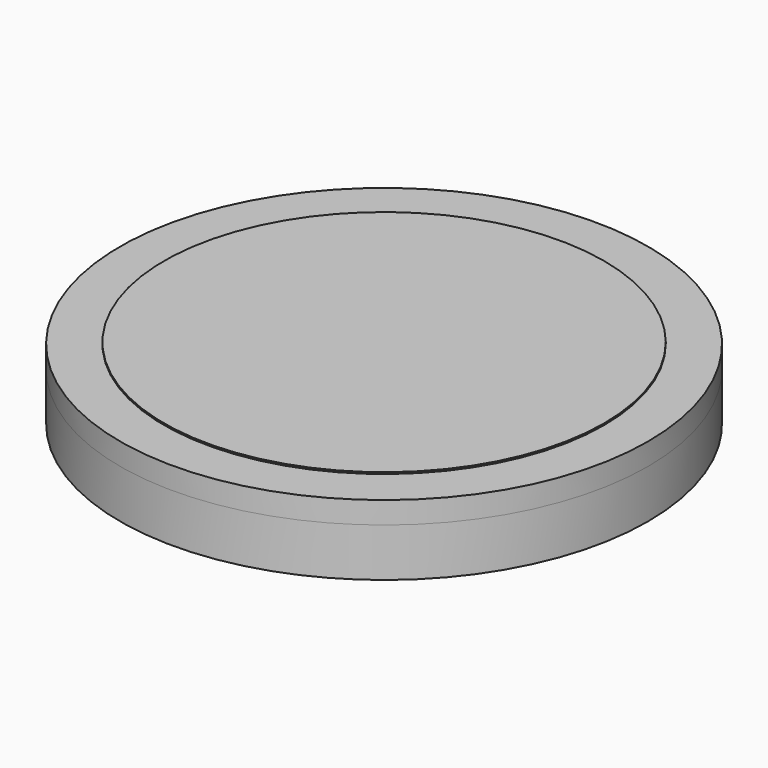
from build123d import *

# Parameters (mm, degrees)
F0_R     = 120
F0_R_2   = 100
F1_DEPTH = 9
F2_DEPTH = 4
F3_DEPTH = 13
F4_DEPTH = 9
F5_DEPTH = 10
F6_R     = 100
F7_DEPTH = 0.75


with BuildPart() as f1:
    # F0 (on Top) → F1 (new body)
    with BuildSketch(Plane.XY):
        Circle(F0_R)
        Circle(F0_R_2, mode=Mode.SUBTRACT)
    extrude(amount=-F1_DEPTH)

    # F0 (on Top) → F3 (join)
    with BuildSketch(Plane.XY):
        Circle(F0_R)
        Circle(F0_R_2, mode=Mode.SUBTRACT)
    extrude(amount=F3_DEPTH)



with BuildPart() as f2:
    # F0 (on Top) → F2 (new body)
    with BuildSketch(Plane.XY):
        Circle(F0_R_2)
    extrude(amount=F2_DEPTH)


with BuildPart() as f1_1:
    add(f1.part)
    # F4 (add): a face of the model
    f4_faces = [f2.part.faces().sort_by_distance(p)[0] for p in [
        (0, 0, 4),
    ]]
    extrude(f4_faces, amount=F4_DEPTH)


with BuildPart() as f5:
    # F5 (new): a face of the model
    f5_faces = [f1_1.part.faces().sort_by_distance(p)[0] for p in [
        (0, 0, 13),
    ]]
    extrude(f5_faces, amount=F5_DEPTH)


with BuildPart() as f7:
    # F6 (on face) → F7 (new body)
    with BuildSketch(Plane.XY.offset(23)):
        Circle(F6_R)
    extrude(amount=F7_DEPTH)


solid = Compound([f2.part, f1_1.part, f5.part, f7.part])
